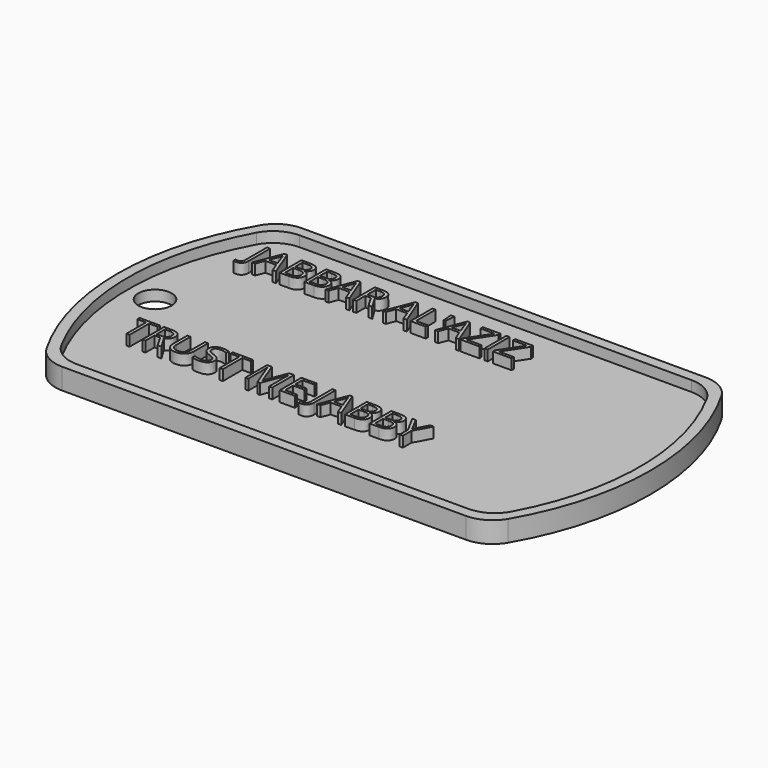
from build123d import *

# Parameters (mm, degrees)
F1_DEPTH     = 1
F3_DEPTH     = 1
F4_R         = 1.5875
F5_DEPTH     = 1
F6_TEXT_SIZE = 3.6260675794
F7_DEPTH     = 1


# Not quite as in the source:
# - Text() gives the source's letters only with a copy of the font that has no kerning and outlines rounded to 1/6400 em; it was checked with that copy


with BuildPart() as f1:
    # F0 (on Top) → F1 (new body)
    with BuildSketch(Plane.XY):
        with BuildLine():
            ThreePointArc((-19.2474145991, 14.2875), (-20.8349145991, 13.862130657), (-21.9970452561, 12.7))
            ThreePointArc((-21.9970452561, 12.7), (-25.4, 0), (-21.9970452561, -12.7))
            ThreePointArc((-21.9970452561, -12.7), (-20.8349145991, -13.862130657), (-19.2474145991, -14.2875))
            Line((-19.2474145991, -14.2875), (19.2474145991, -14.2875))
            ThreePointArc((19.2474145991, -14.2875), (20.8349145991, -13.862130657), (21.9970452561, -12.7))
            ThreePointArc((21.9970452561, -12.7), (25.4, 0), (21.9970452561, 12.7))
            ThreePointArc((21.9970452561, 12.7), (20.8349145991, 13.862130657), (19.2474145991, 14.2875))
            Line((19.2474145991, 14.2875), (-19.2474145991, 14.2875))
        make_face()
    extrude(amount=F1_DEPTH)

    # F2 (on face) → F3 (join)
    with BuildSketch(Plane.XY.offset(1)):
        with BuildLine():
            Line((19.2474145991, 14.2875), (-19.2474145991, 14.2875))
            ThreePointArc((-19.2474145991, 14.2875), (-20.8349145991, 13.862130657), (-21.9970452561, 12.7))
            ThreePointArc((-21.9970452561, 12.7), (-25.4, 0), (-21.9970452561, -12.7))
            ThreePointArc((-21.9970452561, -12.7), (-20.8349145991, -13.862130657), (-19.2474145991, -14.2875))
            Line((-19.2474145991, -14.2875), (19.2474145991, -14.2875))
            ThreePointArc((19.2474145991, -14.2875), (20.8349145991, -13.862130657), (21.9970452561, -12.7))
            ThreePointArc((21.9970452561, -12.7), (25.4, 0), (21.9970452561, 12.7))
            ThreePointArc((21.9970452561, 12.7), (20.8349145991, 13.862130657), (19.2474145991, 14.2875))
        make_face()
        with BuildLine():
            ThreePointArc((-21.4526124879, 11.6252061249), (-20.2856017842, 12.8404540819), (-18.6611352482, 13.2875))
            Line((-18.6611352482, 13.2875), (18.6611352482, 13.2875))
            ThreePointArc((18.6611352482, 13.2875), (20.2856017842, 12.8404540819), (21.4526124879, 11.6252061249))
            ThreePointArc((21.4526124879, 11.6252061249), (24.4, 0), (21.4526124879, -11.6252061249))
            ThreePointArc((21.4526124879, -11.6252061249), (20.2856017842, -12.8404540819), (18.6611352482, -13.2875))
            Line((18.6611352482, -13.2875), (-18.6611352482, -13.2875))
            ThreePointArc((-18.6611352482, -13.2875), (-20.2856017842, -12.8404540819), (-21.4526124879, -11.6252061249))
            ThreePointArc((-21.4526124879, -11.6252061249), (-24.4, 0), (-21.4526124879, 11.6252061249))
        make_face(mode=Mode.SUBTRACT)
    extrude(amount=F3_DEPTH)

    # F4 (on face) → F5 (cut)
    with BuildSketch(Plane.XY.offset(1)):
        with Locations((-21.821282804, 0)):
            Circle(F4_R)
    extrude(amount=-F5_DEPTH, mode=Mode.SUBTRACT)

    # F6 (on face) → F7 (join)
    with BuildSketch(Plane.XY.offset(1)):
        with Locations((-19.6815822273, 7.6558343135)):
            Text("JABBAR AL'AZIZ", F6_TEXT_SIZE, font='Open Sans', text_align=(TextAlign.LEFT, TextAlign.BOTTOM))
        with Locations((-19.6815822273, -7.1385214105)):
            Text('TRUST ME JABBY', F6_TEXT_SIZE, font='Open Sans', text_align=(TextAlign.LEFT, TextAlign.BOTTOM))
    extrude(amount=F7_DEPTH)


solid = f1.part
